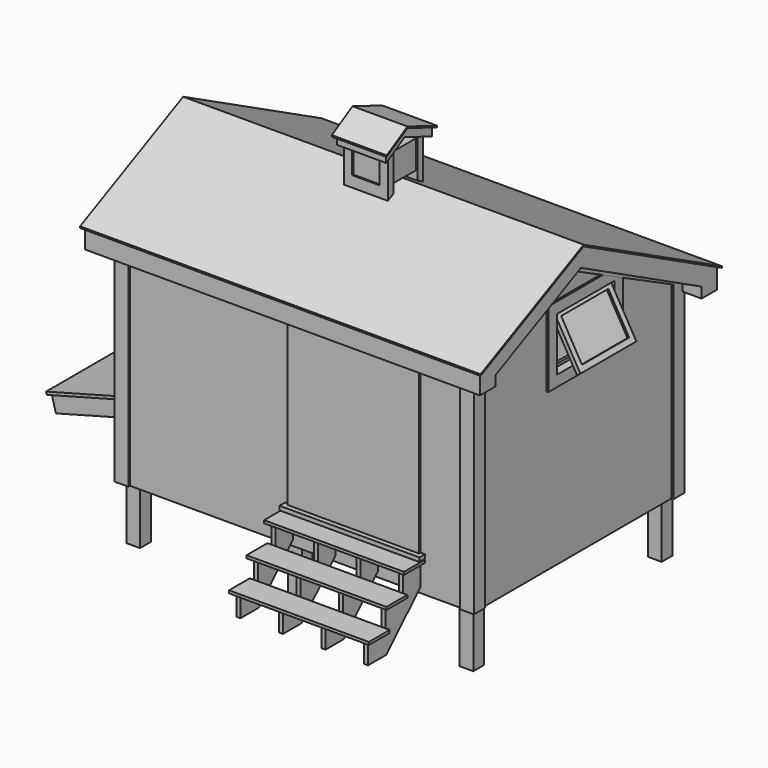
from build123d import *

# Parameters (mm, degrees)
F1_DEPTH       = 3657.6
F3_DEPTH       = 177.8
F5_DEPTH       = 152.4
F6_T           = 101.6
F6_T3_DEPTH    = 3530.6
F6_T5_DEPTH    = 228.6
F6_T7_DEPTH    = 228.6
F6_T9_DEPTH    = 294.3465935833
F6_T11_DEPTH   = 1301.2627674272
F6_T13_DEPTH   = 1775.2993979929
F6_T15_DEPTH   = 301.0795529101
F6_T17_DEPTH   = 355.6
F6_T19_DEPTH   = 1775.2993979929
F6_T21_DEPTH   = 1301.2627674272
F6_T23_DEPTH   = 381
F8_DEPTH       = 19.05
F10_DEPTH      = 19.05
F11_W          = 3073.4
F11_H          = 1854.2
F12_DEPTH      = 19.05
F13_W          = 3073.4
F13_H          = 1600.2
F14_DEPTH      = 19.05
F16_DEPTH      = 25.4
F16_DEPTH_BACK = 3683
F17_W          = 863.6
F17_H          = 698.5
F18_DEPTH      = 17.78
F19_W          = 660.4
F19_H          = 495.3
F20_DEPTH      = 76.2
F21_W          = 1219.2
F21_H          = 1524
F22_DEPTH      = 17.78
F23_W          = 609.6
F23_H          = 444.5
F24_DEPTH      = 76.2
F25_W          = 1168.4
F25_H          = 1651
F26_DEPTH      = 17.78
F30_DEPTH      = 508
F32_DEPTH      = 25.4
F32_DEPTH_BACK = 1041.4
F34_W          = 406.4
F34_H          = 406.4
F35_DEPTH      = 632.46
F37_DEPTH      = 25.4
F37_DEPTH_BACK = 431.8
F39_DEPTH      = 25.4
F39_DEPTH_BACK = 482.6
F40_W          = 279.4
F40_H          = 260.0175112007
F41_DEPTH      = 12.7
F42_W          = 279.4
F42_H          = 260.0175112007
F43_DEPTH      = 12.7
F45_DEPTH      = 152.4
F47_DEPTH      = 152.4
F48_W          = 254
F48_H          = 241.3
F49_DEPTH      = 12.7
F50_W          = 254
F50_H          = 241.3
F51_DEPTH      = 12.7
F55_DEPTH      = 609.6
F56_W          = 355.6
F56_H          = 599.7440126281
F57_DEPTH      = 609.6
F58_W          = 241.3
F58_H          = 25.4
F59_DEPTH      = 38.1
F59_DEPTH_BACK = 1257.3
F60_W          = 63.5
F60_H          = 38.1
F61_DEPTH      = 647.7
F61_DEPTH_BACK = 647.7
F64_DEPTH      = 647.7
F65_W          = 546.1
F65_H          = 386.3676515813
F66_DEPTH      = 19.05
F67_W          = 127
F67_H          = 127
F67_H_2        = 123.2156306505
F68_DEPTH      = 508


# Not quite as in the source:
# - a shell that OpenCascade refuses in one call is made with other operations: the cavity is built on its own and cut out


with BuildPart() as f1:
    # F0 (on Right) → F1 (new body)
    with BuildSketch(Plane.YZ):
        Polygon((-152.4, 2108.2), (-152.4, 1905), (0, 1905), (0, 0), (2438.4, 0), (2438.4, 1651), (2590.8, 1651), (2590.8, 1854.2), (1016, 2667), align=None)
    extrude(amount=F1_DEPTH)

    # F2 (on face) → F3 (cut)
    with BuildSketch(Plane.YZ.offset(3657.6)):
        Polygon((25.4, 1905), (0, 1905), (0, 0), (2438.4, 0), (2438.4, 1651), (2413, 1651), (2413, 1748.8795529101), (1016, 2469.9118109746), (25.4, 1996.1465935833), align=None)
    extrude(amount=-F3_DEPTH, mode=Mode.SUBTRACT)

    # F4 (on face) → F5 (cut)
    with BuildSketch(Plane(origin=(0, 0, 0), x_dir=(0, -1, 0), z_dir=(-1, 0, 0))):
        Polygon((-2413, 1651), (-2438.4, 1651), (-2438.4, 0), (0, 0), (0, 1905), (-25.4, 1905), (-25.4, 1996.1465935833), (-1016, 2469.9118109746), (-2413, 1748.8795529101), align=None)
    extrude(amount=-F5_DEPTH, mode=Mode.SUBTRACT)

    # F6: shell of thickness 101.6, made by hand


with BuildPart() as f6_core1:
    # F6_t2: copy of F1
    add(f1.part)

    # the walls: a layer under each face that stays
    f6_faces = [f6_core1.faces().sort_by_distance(p)[0] for p in [
        (1828.8, 431.8, 2387.6),
        (3657.6, 304.8, 2159),
        (1828.8, 2590.8, 1752.6),
        (1828.8, 2501.9, 1651),
        (152.4, 1219.2, 1234.9559054873),
        (76.2, 1714.5, 2109.3956819424),
        (76.2, 520.7, 2233.029202279),
        (76.2, 25.4, 1950.5732967917),
        (1816.1, 0, 952.5),
        (76.2, 2413, 1699.939776455),
        (3479.8, 1219.2, 1234.9559054873),
        (1816.1, 2438.4, 825.5),
        (3568.7, 2413, 1699.939776455),
        (3568.7, 1714.5, 2109.3956819424),
        (3568.7, 520.7, 2233.029202279),
        (3568.7, 25.4, 1950.5732967917),
        (1828.8, -63.5, 1905),
        (0, 304.8, 2159),
        (1828.8, -152.4, 2006.6),
        (1828.8, 1803.4, 2260.6),
    ]]
    thicken(f6_faces, amount=-F6_T, mode=Mode.SUBTRACT)

    # F6_s4 → F6_t3 (cut)
    with BuildSketch(Plane.YZ.offset(50.8)):
        Polygon((2439.416, 1649.984), (2438.4, 1752.6), (2336.8, 1752.6), (2336.8, 1651), align=None)
        Polygon((-1.016, 1903.984), (101.6, 1905), (101.6, 2006.6), (0, 2006.6), align=None)
    extrude(amount=F6_T3_DEPTH, mode=Mode.SUBTRACT)

    # F6_s6 → F6_t5 (cut)
    with BuildSketch(Plane.XZ.offset(-2540)):
        Polygon((3480.816, 1649.984), (3479.8, 1752.6), (3378.2, 1752.6), (3378.2, 1651), align=None)
        Polygon((151.384, 1649.984), (152.4, 1752.6), (254, 1752.6), (254, 1651), align=None)
    extrude(amount=F6_T5_DEPTH, mode=Mode.SUBTRACT)

    # F6_s8 → F6_t7 (cut)
    with BuildSketch(Plane.XZ.offset(-127)):
        Polygon((151.384, 1903.984), (254, 1905), (254, 2006.6), (152.4, 2006.6), align=None)
        Polygon((3480.816, 1903.984), (3378.2, 1905), (3378.2, 2006.6), (3479.8, 2006.6), align=None)
    extrude(amount=F6_T7_DEPTH, mode=Mode.SUBTRACT)

    # F6_s10 → F6_t9 (cut)
    with BuildSketch(Plane.XY.offset(1803.4)):
        Polygon((151.384, 26.416), (254, 25.4), (254, -76.2), (152.4, -76.2), align=None)
        Polygon((3480.816, 26.416), (3378.2, 25.4), (3378.2, -76.2), (3479.8, -76.2), align=None)
    extrude(amount=F6_T9_DEPTH, mode=Mode.SUBTRACT)

    # F6_s12 → F6_t11 (cut)
    with BuildSketch(Plane(origin=(0, 705.9765295073, 337.6409488948), x_dir=(1, 0, 0), z_dir=(0, 0.9021342216, 0.4314554973))):
        Polygon((151.384, -1788.8171838414), (254, -1789.8331838414), (254, -1891.4331838414), (152.4, -1891.4331838414), align=None)
    extrude(amount=F6_T11_DEPTH, mode=Mode.SUBTRACT)

    # F6_s14 → F6_t13 (cut)
    with BuildSketch(Plane(origin=(0, -294.6390421942, 152.0717637132), x_dir=(1, 0, 0), z_dir=(0, 0.8886206571, -0.4586429198))):
        Polygon((151.384, -2659.7798628224), (254, -2660.7958628224), (254, -2762.3958628224), (152.4, -2762.3958628224), align=None)
    extrude(amount=F6_T13_DEPTH, mode=Mode.SUBTRACT)

    # F6_s16 → F6_t15 (cut)
    with BuildSketch(Plane.XY.offset(1549.4)):
        Polygon((151.384, 2411.984), (254, 2413), (254, 2514.6), (152.4, 2514.6), align=None)
        Polygon((3480.816, 2411.984), (3378.2, 2413), (3378.2, 2514.6), (3479.8, 2514.6), align=None)
    extrude(amount=F6_T15_DEPTH, mode=Mode.SUBTRACT)

    # F6_s18 → F6_t17 (cut)
    with BuildSketch(Plane.YZ.offset(-101.6)):
        Polygon((1015.9723775788, 2468.0924040179), (1062.5981206487, 2560.1956697314), (1017.722341879, 2583.3573619996), (972.1641214739, 2561.5686478928), align=None)
        Polygon((2411.5180187935, 1747.9767143225), (2459.5981206487, 1839.1634116669), (2514.6, 1810.7753449049), (2514.6, 1748.8795529101), align=None)
        Polygon((26.8543587853, 1995.2300252141), (-18.4358785261, 2087.8034305015), (-76.2, 2060.1771115357), (-76.2, 1996.1465935833), align=None)
    extrude(amount=F6_T17_DEPTH, mode=Mode.SUBTRACT)

    # F6_s20 → F6_t19 (cut)
    with BuildSketch(Plane(origin=(0, 1282.9286753193, -662.1567356487), x_dir=(1, 0, 0), z_dir=(0, -0.8886206571, 0.4586429198))):
        Polygon((3480.816, 2659.7798628224), (3378.2, 2660.7958628224), (3378.2, 2762.3958628224), (3479.8, 2762.3958628224), align=None)
    extrude(amount=F6_T19_DEPTH, mode=Mode.SUBTRACT)

    # F6_s22 → F6_t21 (cut)
    with BuildSketch(Plane(origin=(0, 1879.8902033437, 899.0779233383), x_dir=(1, 0, 0), z_dir=(0, -0.9021342216, -0.4314554973))):
        Polygon((3480.816, 1788.8171838414), (3378.2, 1789.8331838414), (3378.2, 1891.4331838414), (3479.8, 1891.4331838414), align=None)
    extrude(amount=F6_T21_DEPTH, mode=Mode.SUBTRACT)

    # F6_s24 → F6_t23 (cut)
    with BuildSketch(Plane.YZ.offset(3378.2)):
        Polygon((2411.5180187935, 1747.9767143225), (2514.6, 1748.8795529101), (2514.6, 1810.7753449049), (2459.5981206487, 1839.1634116669), align=None)
        Polygon((1015.9723775788, 2468.0924040179), (1062.5981206487, 2560.1956697314), (1017.722341879, 2583.3573619996), (972.1641214739, 2561.5686478928), align=None)
        Polygon((26.8543587853, 1995.2300252141), (-18.4358785261, 2087.8034305015), (-76.2, 2060.1771115357), (-76.2, 1996.1465935833), align=None)
    extrude(amount=F6_T23_DEPTH, mode=Mode.SUBTRACT)


with BuildPart() as f1_1:
    add(f1.part)

    # what is left inside the walls is the cavity
    f6_cavity = [f6_core1.part.solids().sort_by_distance(p)[0] for p in [
        (2336.8, 1219.2, 1.016),
    ]]
    add(f6_cavity, mode=Mode.SUBTRACT)

    # F7 (on face) → F8 (cut)
    with BuildSketch(Plane.YZ.offset(3479.8)):
        Polygon((127, 1974.3492589935), (127, 0), (2311.4, 0), (2311.4, 1748.8795529101), (1016, 2399.523172037), align=None)
    extrude(amount=-F8_DEPTH, mode=Mode.SUBTRACT)

    # F9 (on face) → F10 (cut)
    with BuildSketch(Plane(origin=(152.4, 0, 0), x_dir=(0, -1, 0), z_dir=(-1, 0, 0))):
        Polygon((-2311.4, 1748.8795529101), (-2311.4, 0), (-127, 0), (-127, 1974.3492589935), (-1016, 2399.523172037), align=None)
    extrude(amount=-F10_DEPTH, mode=Mode.SUBTRACT)

    # F11 (on face) → F12 (cut)
    with BuildSketch(Plane.XZ):
        with Locations((1816.1, 927.1)):
            Rectangle(F11_W, F11_H)
    extrude(amount=-F12_DEPTH, mode=Mode.SUBTRACT)

    # F13 (on face) → F14 (cut)
    with BuildSketch(Plane(origin=(0, 2438.4, 0), x_dir=(-1, 0, 0), z_dir=(0, 1, 0))):
        with Locations((-1816.1, 800.1)):
            Rectangle(F13_W, F13_H)
    extrude(amount=-F14_DEPTH, mode=Mode.SUBTRACT)

    # F15 (on face) → F16 (join, two sides)
    with BuildSketch(Plane.YZ.offset(3657.6)) as f16_sk:
        Polygon((2616.2, 1841.0903225806), (1016, 2667), (-177.8, 2096.052173913), (-177.8, 2081.9744461255), (1016, 2652.9222722125), (2616.2, 1827.0125947931), align=None)
    extrude(amount=F16_DEPTH)
    extrude(f16_sk.sketch, amount=-F16_DEPTH_BACK)

    # F17 (on face) → F18 (join)
    with BuildSketch(Plane.YZ.offset(3460.75)):
        with Locations((1295.4, 1809.75)):
            Rectangle(F17_W, F17_H)
    extrude(amount=F18_DEPTH)

    # F19 (on face) → F20 (cut)
    with BuildSketch(Plane.YZ.offset(3478.53)):
        with Locations((1295.4, 1809.75)):
            Rectangle(F19_W, F19_H)
    extrude(amount=-F20_DEPTH, mode=Mode.SUBTRACT)

    # F21 (on face) → F22 (join)
    with BuildSketch(Plane.XZ.offset(-19.05)):
        with Locations((2362.2, 1092.2)):
            Rectangle(F21_W, F21_H)
    extrude(amount=F22_DEPTH)

    # F23 (on face) → F24 (cut)
    with BuildSketch(Plane.YZ.offset(3402.33)):
        with Locations((1295.4, 1809.75)):
            Rectangle(F23_W, F23_H)
    extrude(amount=-F24_DEPTH, mode=Mode.SUBTRACT)

    # F25 (on face) → F26 (join)
    with BuildSketch(Plane(origin=(171.45, 0, 0), x_dir=(0, -1, 0), z_dir=(-1, 0, 0))):
        with Locations((-1219.2, 1269.223172037)):
            Rectangle(F25_W, F25_H)
    extrude(amount=F26_DEPTH)

    # F29 (on plane+point) → F30 (join, symmetric)
    with BuildSketch(Plane.XZ.offset(-1219.2)):
        Polygon((171.45, 208.8510671601), (171.45, 392.923172037), (-1006.2067674116, 77.370992248), (-960.1887411924, -94.3706196662), align=None)
    extrude(amount=F30_DEPTH, both=True)

    # F31 (on face) → F32 (join, two sides)
    with BuildSketch(Plane.XZ.offset(-711.2)) as f32_sk:
        Polygon((171.45, 366.6271570546), (171.45, 392.923172037), (-1030.7412833994, 70.7969885024), (-1024.1672796538, 46.2624725146), align=None)
    extrude(amount=F32_DEPTH)
    extrude(f32_sk.sketch, amount=-F32_DEPTH_BACK)

    # F34 (on plane+point) → F35 (join)
    with BuildSketch(Plane(origin=(0, 0, 2399.523172037), x_dir=(1, 0, 0), z_dir=(0, 0, -1))):
        with Locations((1828.8, -1016)):
            Rectangle(F34_W, F34_H)
    extrude(amount=-F35_DEPTH)

    # F36 (on face) → F37 (join, two sides)
    with BuildSketch(Plane.YZ.offset(2032)) as f37_sk:
        Polygon((976.217410692, 3126.3322580903), (762, 3002.6537783621), (762, 2907.2870922648), (976.217410692, 3030.965571993), (1294.733662445, 2907.2870922648), (1294.733662445, 3002.6537783621), align=None)
    extrude(amount=F37_DEPTH)
    extrude(f37_sk.sketch, amount=-F37_DEPTH_BACK)

    # F38 (on face) → F39 (join, two sides)
    with BuildSketch(Plane.YZ.offset(2057.4)) as f39_sk:
        Polygon((1320.133662445, 2992.7910684759), (976.217410692, 3126.3322580903), (736.6, 2987.9890815247), (736.6, 2974.3652692251), (976.217410692, 3112.7084457907), (1320.133662445, 2979.1672561763), align=None)
    extrude(amount=F39_DEPTH)
    extrude(f39_sk.sketch, amount=-F39_DEPTH_BACK)

    # F40 (on face) → F41 (cut)
    with BuildSketch(Plane.YZ.offset(2032)):
        with Locations((1016, 2806.6077303393)):
            Rectangle(F40_W, F40_H)
    extrude(amount=-F41_DEPTH, mode=Mode.SUBTRACT)

    # F42 (on face) → F43 (cut)
    with BuildSketch(Plane(origin=(1625.6, 0, 0), x_dir=(0, -1, 0), z_dir=(-1, 0, 0))):
        with Locations((-1016, 2806.6077303393)):
            Rectangle(F42_W, F42_H)
    extrude(amount=-F43_DEPTH, mode=Mode.SUBTRACT)

    # F44 (on face) → F45 (cut)
    with BuildSketch(Plane.YZ.offset(2032)):
        Polygon((876.3, 2973.2782280332), (876.3, 2936.6164859397), (1155.7, 2936.6164859397), (1155.7, 2961.2732606553), (976.217410692, 3030.965571993), align=None)
        Polygon((1155.7, 2676.598974739), (876.3, 2676.598974739), (876.3, 2600.1869565217), (1016, 2667), (1155.7, 2594.8967741935), align=None)
    extrude(amount=-F45_DEPTH, mode=Mode.SUBTRACT)

    # F46 (on face) → F47 (cut)
    with BuildSketch(Plane(origin=(1625.6, 0, 0), x_dir=(0, -1, 0), z_dir=(-1, 0, 0))):
        Polygon((-1155.7, 2961.2732606553), (-1155.7, 2936.6164859397), (-876.3, 2936.6164859397), (-876.3, 2973.2782280332), (-976.217410692, 3030.965571993), align=None)
        Polygon((-1155.7, 2594.8967741935), (-1016, 2667), (-876.3, 2600.1869565217), (-876.3, 2676.598974739), (-1155.7, 2676.598974739), align=None)
    extrude(amount=-F47_DEPTH, mode=Mode.SUBTRACT)

    # F48 (on face) → F49 (cut)
    with BuildSketch(Plane.XZ.offset(-812.8)):
        with Locations((1828.8, 2792.3675361736)):
            Rectangle(F48_W, F48_H)
    extrude(amount=-F49_DEPTH, mode=Mode.SUBTRACT)

    # F50 (on face) → F51 (cut)
    with BuildSketch(Plane(origin=(0, 1219.2, 0), x_dir=(-1, 0, 0), z_dir=(0, 1, 0))):
        with Locations((-1828.8, 2792.3675361736)):
            Rectangle(F50_W, F50_H)
    extrude(amount=-F51_DEPTH, mode=Mode.SUBTRACT)

    # F54 (on plane+point) → F55 (join, symmetric)
    with BuildSketch(Plane.YZ.offset(2362.2)):
        Polygon((19.05, 55.88), (19.05, 259.08), (-184.15, 259.08), (-184.15, 55.88), (-387.35, 55.88), (-387.35, -147.32), (-590.55, -147.32), (-590.55, -340.6640126281), (-377.4940126281, -340.6640126281), align=None)
    extrude(amount=F55_DEPTH, both=True)

    # F56 (on face) → F57 (cut, through all)
    with BuildSketch(Plane.XZ.offset(590.55)):
        with Locations((1968.5, -40.7920063141)):
            Rectangle(F56_W, F56_H)
        with Locations((2362.2, -40.7920063141)):
            Rectangle(F56_W, F56_H)
        with Locations((2755.9, -40.7920063141)):
            Rectangle(F56_W, F56_H)
    extrude(amount=-F57_DEPTH, mode=Mode.SUBTRACT)

    # F58 (on face) → F59 (join, two sides)
    with BuildSketch(Plane.YZ.offset(2971.8)) as f59_sk:
        with Locations((-101.6, 271.78)):
            Rectangle(F58_W, F58_H)
        with Locations((-304.8, 68.58)):
            Rectangle(F58_W, F58_H)
        with Locations((-508, -134.62)):
            Rectangle(F58_W, F58_H)
    extrude(amount=F59_DEPTH)
    extrude(f59_sk.sketch, amount=-F59_DEPTH_BACK)

    # F60 (on plane+point) → F61 (join, two sides)
    with BuildSketch(Plane.YZ.offset(2362.2)) as f61_sk:
        with Locations((-12.7, 311.15)):
            Rectangle(F60_W, F60_H)
    extrude(amount=F61_DEPTH)
    extrude(f61_sk.sketch, amount=-F61_DEPTH_BACK)

    # F63 (on offset) → F64 (join)
    with BuildSketch(Plane.XZ.offset(-1619.25)):
        Polygon((3440.43, 2063.75), (3407.4344321158, 2044.7), (3655.0844321158, 1615.7576175056), (3688.08, 1634.8076175056), align=None)
    extrude(amount=F64_DEPTH)

    # F65 (on face) → F66 (cut)
    with BuildSketch(Plane(origin=(3473.9524635301, 0, 2005.687389971), x_dir=(0, 1, 0), z_dir=(0.8660254038, 0, 0.5))):
        with Locations((1295.4, -184.2712471492)):
            Rectangle(F65_W, F65_H)
    extrude(amount=-F66_DEPTH, mode=Mode.SUBTRACT)

    # F67 (on face) → F68 (join)
    with BuildSketch(Plane(origin=(0, 0, 0), x_dir=(1, 0, 0), z_dir=(0, 0, -1))):
        with Locations((273.05, -127)):
            Rectangle(F67_W, F67_H)
        with Locations((1771.1507806778, -125.1078153253)):
            Rectangle(F67_W, F67_H_2)
        with Locations((3359.15, -125.1078153253)):
            Rectangle(F67_W, F67_H_2)
        with Locations((3352.8, -2315.5175914764)):
            Rectangle(F67_W, F67_H)
        with Locations((1786.0860357285, -2315.5175914764)):
            Rectangle(F67_W, F67_H)
        with Locations((273.05, -2315.5175914764)):
            Rectangle(F67_W, F67_H)
    extrude(amount=F68_DEPTH)


solid = f1_1.part
